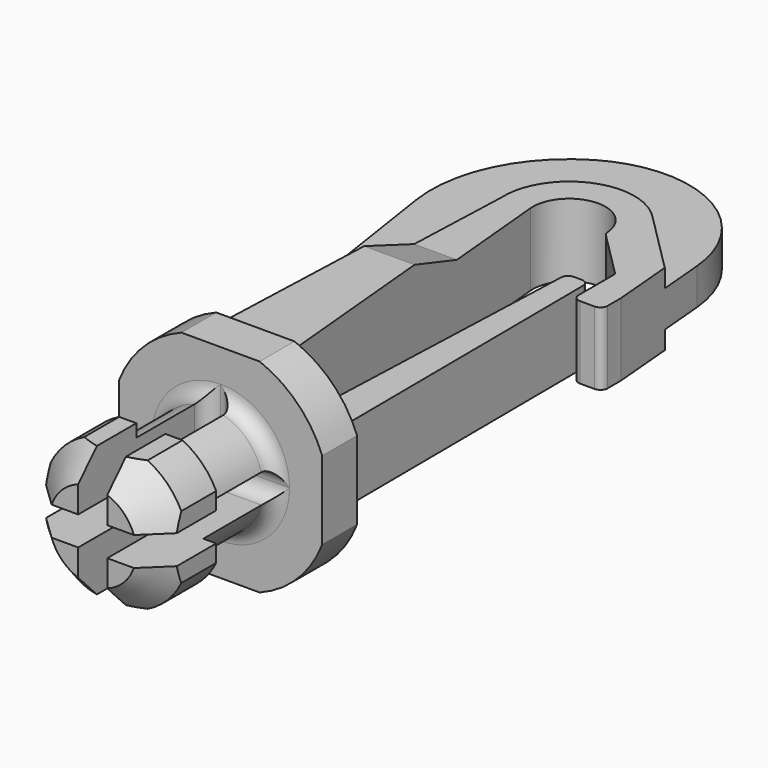
from build123d import *

# Parameters (mm, degrees)
F1_DEPTH  = 1.25
F3_DEPTH  = 4
F4_R      = 7.5
F5_DEPTH  = 3
F7_DEPTH  = 2.5
F9_DEPTH  = 12.5
F10_R     = 3.75
F11_DEPTH = 6
F12_R     = 5
F13_DEPTH = 5
F14_SIZE  = 2
F16_DEPTH = 11
F17_R     = 8
F18_R     = 0.5
F19_W     = 20
F19_H     = 20
F19_W_2   = 9
F19_H_2   = 9
F20_DEPTH = 11.001
F21_R     = 0.99999
F22_W     = 20
F22_H     = 20
F22_W_2   = 14
F22_H_2   = 14
F23_DEPTH = 3


# Not quite as in the source:
# - a fillet or chamfer is up to 0.001 mm smaller than in the source, because OpenCascade refuses the exact size


with BuildPart() as f1:
    # F0 (on Top) → F1 (new body, symmetric)
    with BuildSketch(Plane.XY):
        with BuildLine():
            ThreePointArc((-2.4892601961, 26.7685185185), (-0.1158652446, 29.4973136057), (2.5, 27))
            Line((2.5, 27), (7.8501893912, 21.6498106088))
            Line((7.8501893912, 21.6498106088), (6.8018767371, 33.6320790747))
            ThreePointArc((6.8018767371, 33.6320790747), (-4.2336746433, 35.5044693553), (-9.391842346, 25.5705604779))
            Line((-9.391842346, 25.5705604779), (-5.5, 0))
            Line((-5.5, 0), (0, 0))
            Line((0, 0), (-2.4892601961, 26.7685185185))
        make_face()
    extrude(amount=F1_DEPTH, both=True)

    # F2 (on Top) → F3 (join, symmetric)
    with BuildSketch(Plane.XY):
        Polygon((-5.5, 0), (0, 0), (-2.4892601961, 26.7685185185), (-4.4892601961, 26.7685185185), align=None)
        with BuildLine():
            Line((-4.4892601961, 26.7685185185), (-2.4892601961, 26.7685185185))
            ThreePointArc((-2.4892601961, 26.7685185185), (-0.1158652446, 29.4973136057), (2.5, 27))
            Line((2.5, 27), (5.8501893912, 23.6498106088))
            Line((5.8501893912, 23.6498106088), (7.8501893912, 21.6498106088))
            Line((7.8501893912, 21.6498106088), (7.4803727359, 25.8768343213))
            Line((7.4803727359, 25.8768343213), (3.1786035286, 30.1786035286))
            ThreePointArc((3.1786035286, 30.1786035286), (-1.8266431422, 31.1073611498), (-4.4892601961, 26.7685185185))
        make_face()
        Polygon((7.8501893912, 21.6498106088), (5.8501893912, 23.6498106088), (5.8501893912, 20), (7.8501893912, 20), align=None)
    extrude(amount=F3_DEPTH, both=True)

    # F4 (on Front) → F5 (join)
    with BuildSketch(Plane.XZ):
        Circle(F4_R)
    extrude(amount=F5_DEPTH)

    # F6 (on Top) → F7 (join, symmetric)
    with BuildSketch(Plane.XY):
        Polygon((3.8501893912, 22), (3, 0), (5.5, 0), (5.3501893912, 22), align=None)
    extrude(amount=F7_DEPTH, both=True)

    # F8 (on Right) → F9 (cut, symmetric)
    with BuildSketch(Plane.YZ):
        Polygon((31.4952242196, 2.5), (31.4952242196, 4), (26.7685185185, 4), (15.4952242196, 4), (19.6164403488, 2.5), align=None)
        Polygon((26.7685185185, -4), (31.4952242196, -4), (31.4952242196, -2.5), (19.6164403488, -2.5), (15.4952242196, -4), align=None)
    extrude(amount=F9_DEPTH, both=True, mode=Mode.SUBTRACT)

    # F10 (on face) → F11 (join)
    with BuildSketch(Plane.XZ.offset(3)):
        Circle(F10_R)
    extrude(amount=F11_DEPTH)

    # F12 (on face) → F13 (join)
    with BuildSketch(Plane.XZ.offset(9)):
        Circle(F12_R)
    extrude(amount=F13_DEPTH)

    # F14
    f14_edges = [f1.edges().sort_by_distance(p)[0] for p in [
        (-5, -14, 0),
    ]]
    chamfer(f14_edges, length=F14_SIZE)

    # F15 (on face) → F16 (cut, through all)
    with BuildSketch(Plane.XZ.offset(14)):
        Polygon((1, 1), (1, 10), (-1, 10), (-1, 1), (-10, 1), (-10, -1), (-1, -1), (-1, -10), (1, -10), (1, -1), (10, -1), (10, 1), align=None)
    extrude(amount=-F16_DEPTH, mode=Mode.SUBTRACT)

    # F17
    f17_edges = [f1.edges().sort_by_distance(p)[0] for p in [
        (6.801877, 33.632079, 0),
    ]]
    fillet(f17_edges, radius=F17_R)

    # F18
    f18_edges = [f1.edges().sort_by_distance(p)[0] for p in [
        (5.850189, 20, 0),
        (7.850189, 20, 0),
        (5.350189, 22, 0),
        (3.850189, 22, 0),
        (2.5, 27, 0),
        (0, 0, 0),
        (5.5, 0, 0),
        (3, 0, 0),
        (-5.5, 0, 0),
    ]]
    fillet(f18_edges, radius=F18_R)

    # F19 (on face) → F20 (cut, through all)
    with BuildSketch(Plane.XZ.offset(3)):
        Rectangle(F19_W, F19_H)
        Rectangle(F19_W_2, F19_H_2, mode=Mode.SUBTRACT)
    extrude(amount=F20_DEPTH, mode=Mode.SUBTRACT)

    # F21 (radius 1 in the source; OpenCascade refuses exactly that, so slightly less here)
    f21_edges = [f1.edges().sort_by_distance(p)[0] for p in [
        (-2.65165, -3, -2.65165),
        (2.65165, -3, -2.65165),
        (2.65165, -3, 2.65165),
        (-2.65165, -3, 2.65165),
        (-1, -3, 2.307104),
        (1, -3, 2.307104),
        (2.307104, -3, 1),
        (-2.307104, -3, 1),
        (-2.307104, -3, -1),
        (2.307104, -3, -1),
        (-1, -3, -2.307104),
        (1, -3, -2.307104),
    ]]
    fillet(f21_edges, radius=F21_R)

    # F22 (on Front) → F23 (cut, through all)
    with BuildSketch(Plane.XZ):
        Rectangle(F22_W, F22_H)
        Rectangle(F22_W_2, F22_H_2, mode=Mode.SUBTRACT)
    extrude(amount=F23_DEPTH, mode=Mode.SUBTRACT)


solid = f1.part
